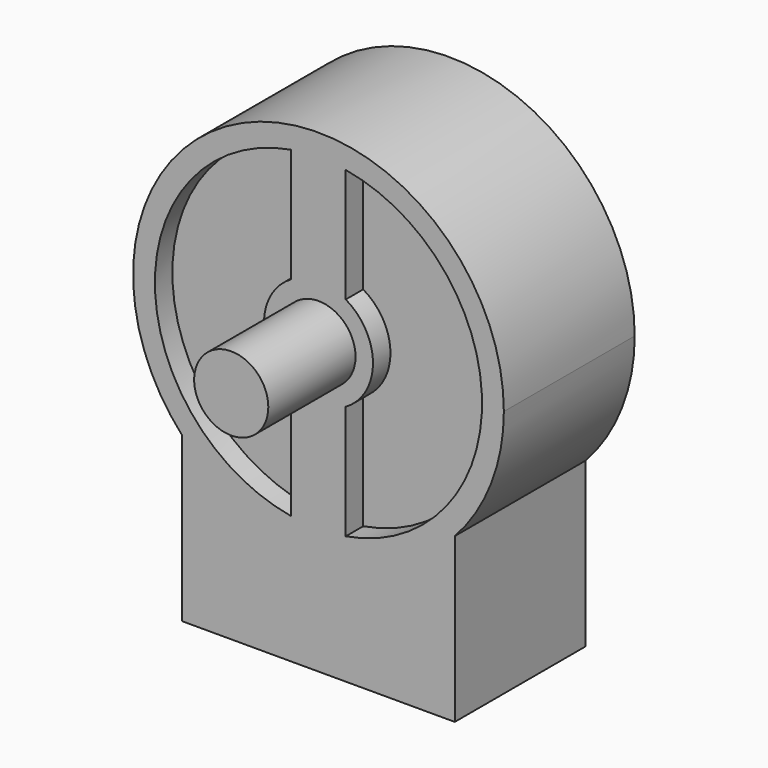
from build123d import *

# Parameters (mm, degrees)
F1_DEPTH = 15
F3_DEPTH = 2
F4_R     = 3.4
F5_DEPTH = 10


# Not quite as in the source:
# - a feature of the source that left no trace in its solid (it failed there, or was rolled back) is left out
# - a pattern or mirror of a feature is missing from the dataset's text; its kind, count and spacing are read off the source's solid


with BuildPart() as f1:
    # F0 (on Front) → F1 (new body)
    with BuildSketch(Plane.XZ):
        with BuildLine():
            ThreePointArc((12.5, -11.5217186218), (15.8350876221, -6.1846584384), (17, 0))
            ThreePointArc((17, 0), (-6.1846584384, 15.8350876221), (-12.5, -11.5217186218))
            ThreePointArc((-12.5, -11.5217186218), (0, -17), (12.5, -11.5217186218))
        make_face()
        with BuildLine():
            ThreePointArc((12.5, -11.5217186218), (0, -17), (-12.5, -11.5217186218))
            Line((-12.5, -11.5217186218), (-12.5, -26.5217186218))
            Line((-12.5, -26.5217186218), (12.5, -26.5217186218))
            Line((12.5, -26.5217186218), (12.5, -11.5217186218))
        make_face()
    extrude(amount=F1_DEPTH)

    # F2 (on face) → F3 (cut)
    with BuildSketch(Plane.XZ.offset(15)):
        with BuildLine():
            Line((-2.5, 4.3301270189), (-2.5, 14.7901994577))
            ThreePointArc((-2.5, 14.7901994577), (-15, 0), (-2.5, -14.7901994577))
            Line((-2.5, -14.7901994577), (-2.5, -4.3301270189))
            ThreePointArc((-2.5, -4.3301270189), (-5, 0), (-2.5, 4.3301270189))
        make_face()
    f3 = extrude(amount=-F3_DEPTH, mode=Mode.SUBTRACT)

    # F3_copies: F3 across plane
    add(f3.mirror(Plane(origin=(0, 0, 0), x_dir=(0, 0, 1), z_dir=(1, 0, 0))), mode=Mode.SUBTRACT)

    # F4 (on face) → F5 (join)
    with BuildSketch(Plane.XZ.offset(15)):
        Circle(F4_R)
    extrude(amount=F5_DEPTH)


solid = f1.part
